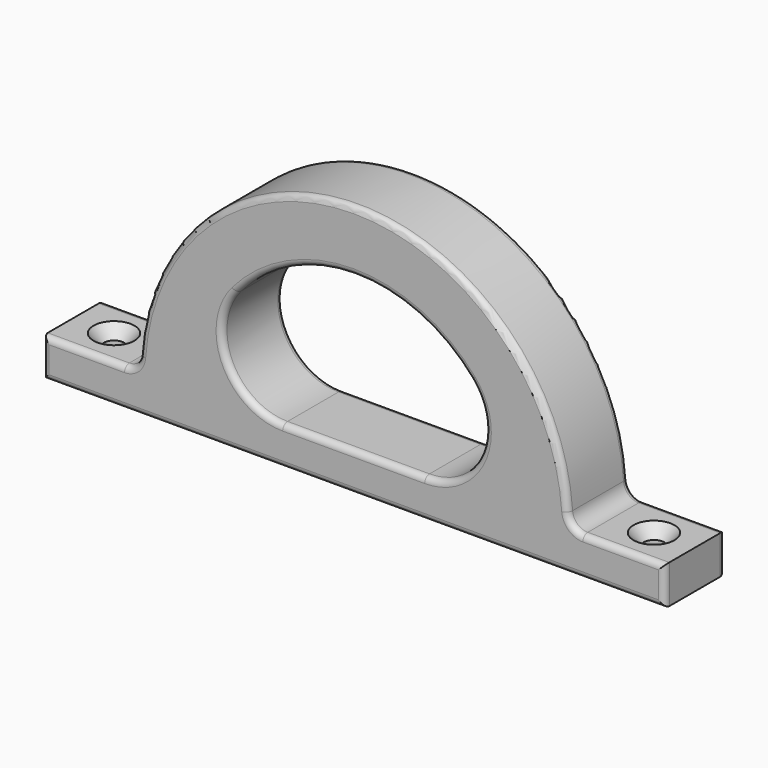
from build123d import *

# Parameters (mm, degrees)
F1_DEPTH       = 25
F2_R           = 20
F3_R           = 5
F5_D           = 6.7564
F5_DEPTH       = 15
F5_CSINK_D     = 13.4874
F5_CSINK_ANGLE = 82
F5_TIP         = 2.0298273432
F6_R           = 2


with BuildPart() as f1:
    # F0 (on Front) → F1 (new body)
    with BuildSketch(Plane.XZ):
        Polygon((-70.8, 12.7), (-102.55, 12.7), (-102.55, 0), (102.55, 0), (102.55, 12.7), (70.8, 12.7), (50.8, 12.7), (-50.8, 12.7), align=None)
        with BuildLine():
            ThreePointArc((70.8, 12.7), (0, 83.5), (-70.8, 12.7))
            Line((-70.8, 12.7), (-50.8, 12.7))
            ThreePointArc((-50.8, 12.7), (0, 63.5), (50.8, 12.7))
            Line((50.8, 12.7), (70.8, 12.7))
        make_face()
    extrude(amount=F1_DEPTH)

    # F2
    f2_edges = [f1.edges().sort_by_distance(p)[0] for p in [
        (50.8, -12.5, 12.7),
        (-50.8, -12.5, 12.7),
    ]]
    fillet(f2_edges, radius=F2_R)

    # F3
    f3_edges = [f1.edges().sort_by_distance(p)[0] for p in [
        (70.8, -12.5, 12.7),
        (-70.8, -12.5, 12.7),
    ]]
    fillet(f3_edges, radius=F3_R)

    # F5
    with Locations(Plane.XY.offset(12.7)):
        with Locations((89.0924562867, -12.5), (-89.0924562867, -12.5)):
            CounterSinkHole(F5_D / 2, F5_CSINK_D / 2, depth=F5_DEPTH, counter_sink_angle=F5_CSINK_ANGLE)
            with Locations((0, 0, -(F5_DEPTH + F5_TIP / 2))):  # 118° drill point
                Cone(0, F5_D / 2, F5_TIP, mode=Mode.SUBTRACT)

    # F6
    f6_edges = [f1.edges().sort_by_distance(p)[0] for p in [
        (-89.092456, -25, 12.7),
        (-72.217975, -25, 14.049721),
        (-102.55, -25, 6.35),
        (0, -25, 83.5),
        (0, -25, 0),
        (72.217975, -25, 14.049721),
        (102.55, -25, 6.35),
        (89.092456, -25, 12.7),
        (0, -25, 12.7),
        (41.585393, -25, 24.325642),
        (-41.585393, -25, 24.325642),
        (0, -25, 63.5),
        (-89.092456, 0, 12.7),
        (-72.217975, 0, 14.049721),
        (-102.55, 0, 6.35),
        (0, 0, 83.5),
        (0, 0, 0),
        (72.217975, 0, 14.049721),
        (102.55, 0, 6.35),
        (89.092456, 0, 12.7),
        (0, 0, 12.7),
        (41.585393, 0, 24.325642),
        (-41.585393, 0, 24.325642),
        (0, 0, 63.5),
    ]]
    fillet(f6_edges, radius=F6_R)


solid = f1.part
